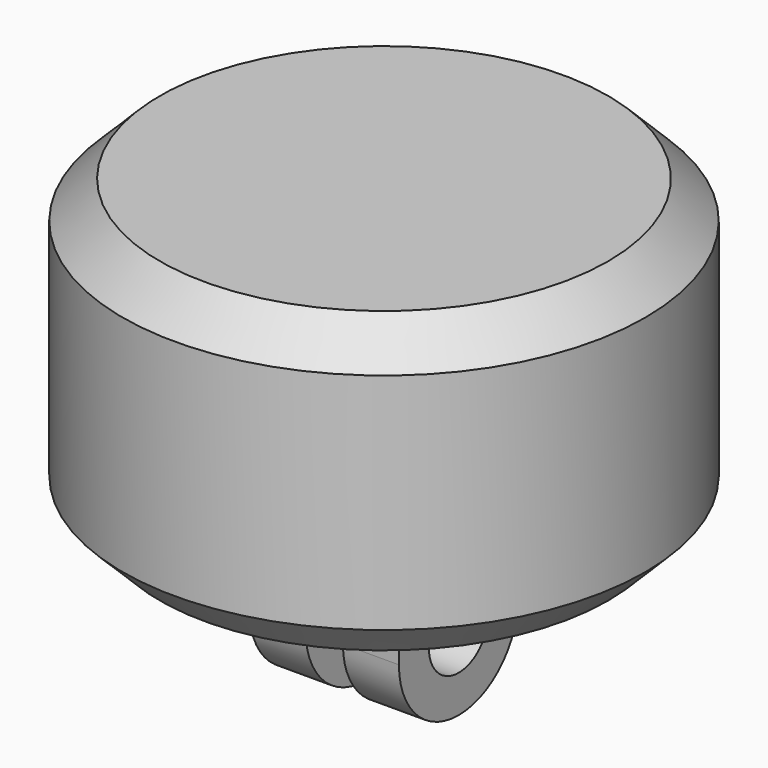
from build123d import *

# Parameters (mm, degrees)
F0_R     = 88.9
F1_DEPTH = 101.6
F2_SIZE  = 12.7
F3_W     = 50.8
F3_H     = 50.8
F4_DEPTH = 50.8
F5_W     = 12.7
F5_H     = 50.8
F6_DEPTH = 50.8
F7_R     = 25.39999
F8_R     = 12.7
F9_DEPTH = 50.8


# Not quite as in the source:
# - a fillet or chamfer is up to 0.001 mm smaller than in the source, because OpenCascade refuses the exact size


with BuildPart() as f1:
    # F0 (on Top) → F1 (new body)
    with BuildSketch(Plane.XY):
        Circle(F0_R)
    extrude(amount=F1_DEPTH)

    # F2
    f2_edges = [f1.edges().sort_by_distance(p)[0] for p in [
        (-88.9, 0, 101.6),
        (-88.9, 0, 0),
    ]]
    chamfer(f2_edges, length=F2_SIZE)

    # F3 (on face) → F4 (join)
    with BuildSketch(Plane(origin=(0, 0, 0), x_dir=(1, 0, 0), z_dir=(0, 0, -1))):
        Rectangle(F3_W, F3_H)
    extrude(amount=F4_DEPTH)

    # F5 (on face) → F6 (cut)
    with BuildSketch(Plane.XZ.offset(25.4)):
        with Locations((0, -25.4)):
            Rectangle(F5_W, F5_H)
    extrude(amount=-F6_DEPTH, mode=Mode.SUBTRACT)

    # F7 (radius 25.4 in the source; OpenCascade refuses exactly that, so slightly less here)
    f7_edges = [f1.edges().sort_by_distance(p)[0] for p in [
        (-15.875, -25.4, -50.8),
        (-15.875, 25.4, -50.8),
        (15.875, 25.4, -50.8),
        (15.875, -25.4, -50.8),
    ]]
    fillet(f7_edges, radius=F7_R)

    # F8 (on face) → F9 (cut, through all)
    with BuildSketch(Plane(origin=(-25.4, 0, 0), x_dir=(0, -1, 0), z_dir=(-1, 0, 0))):
        with Locations((0, -25.4)):
            Circle(F8_R)
    extrude(amount=-F9_DEPTH, mode=Mode.SUBTRACT)


solid = f1.part
